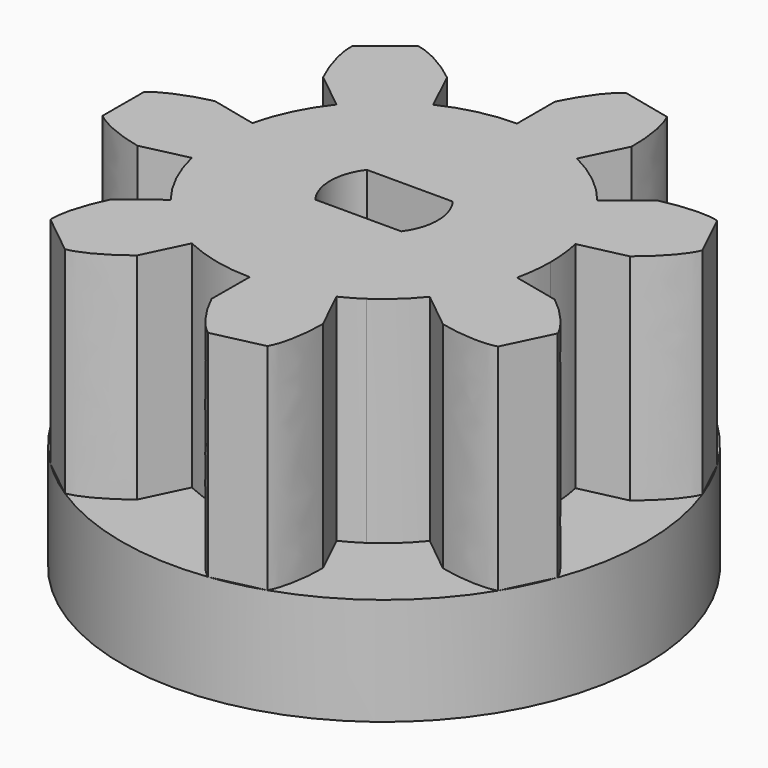
from build123d import *

# Parameters (mm, degrees)
F1_DEPTH        = 10
F2_DEPTH        = 10
F2_COPIES_COUNT = 7
F4_R            = 12.2091154471
F5_DEPTH        = 5


# Not quite as in the source:
# - a pattern or mirror of a feature is missing from the dataset's text; its kind, count and spacing are read off the source's solid


with BuildPart() as f1:
    # F0 (on Top) → F1 (new body)
    with BuildSketch(Plane.XY):
        with BuildLine():
            ThreePointArc((4.3237516011, -6.4317705254), (6.8400137028, -3.6437223475), (7.75, 0))
            ThreePointArc((7.75, 0), (6.5755629687, 4.1017644551), (3.4082008658, 6.9603639889))
            ThreePointArc((3.4082008658, 6.9603639889), (1.7433706712, 7.5513680021), (-0.0120479028, 7.7499906354))
            ThreePointArc((-0.0120479028, 7.7499906354), (-5.6679911875, 5.2854872905), (-7.7319524669, -0.5285934635))
            ThreePointArc((-7.7319524669, -0.5285934635), (-3.4082008658, -6.9603639889), (4.3237516011, -6.4317705254))
        make_face()
        with BuildLine():
            ThreePointArc((-2, -1.5), (-2.5, 0), (-2, 1.5))
            Line((-2, 1.5), (2, 1.5))
            ThreePointArc((2, 1.5), (2.5, 0), (2, -1.5))
            Line((2, -1.5), (-2, -1.5))
        make_face(mode=Mode.SUBTRACT)
    extrude(amount=F1_DEPTH)

    # F0 (on Top) → F2 (join)
    with BuildSketch(Plane.XY):
        with BuildLine():
            ThreePointArc((-0.0120479028, 7.7499906354), (1.7433706712, 7.5513680021), (3.4082008658, 6.9603639889))
            Line((3.4082008658, 6.9603639889), (4.3726173887, 8.9377108908))
            add(Edge.make_bspline(
                [(4.3726173887, 8.9377108908), (4.3837213667, 9.6011226956), (4.2995730436, 10.8287649694), (3.902399388, 11.5686550219)],
                knots=[0, 0, 0, 0, 2.6726339048, 2.6726339048, 2.6726339048, 2.6726339048], degree=3))
            Line((3.902399388, 11.5686550219), (1.5639112325, 12.1085375524))
            add(Edge.make_bspline(
                [(-0.0120479028, 9.9499906354), (0.2687925016, 10.5511288793), (0.8825874647, 11.6176382491), (1.5639112325, 12.1085375524)],
                knots=[0, 0, 0, 0, 2.6726339048, 2.6726339048, 2.6726339048, 2.6726339048], degree=3))
            Line((-0.0120479028, 9.9499906354), (-0.0120479028, 7.7499906354))
        make_face()
    f2 = extrude(amount=F2_DEPTH)

    # F2_copies: F2 ×7 about axis
    f2_copies_axis = Axis((0, 0, 0), (0, 0, 1))
    for i in range(1, F2_COPIES_COUNT):
        add(f2.rotate(f2_copies_axis, i * 360 / F2_COPIES_COUNT))

    # F4 (on face) + F0 (on Top) → F5 (join)
    with BuildSketch(Plane.XY):
        Circle(F4_R)
        with BuildLine():
            ThreePointArc((7.75, 0), (6.8400137028, -3.6437223475), (4.3237516011, -6.4317705254))
            ThreePointArc((4.3237516011, -6.4317705254), (-3.4082008658, -6.9603639889), (-7.7319524669, -0.5285934635))
            ThreePointArc((-7.7319524669, -0.5285934635), (-5.6679911875, 5.2854872905), (-0.0120479028, 7.7499906354))
            ThreePointArc((-0.0120479028, 7.7499906354), (1.7433706712, 7.5513680021), (3.4082008658, 6.9603639889))
            ThreePointArc((3.4082008658, 6.9603639889), (6.5755629687, 4.1017644551), (7.75, 0))
        make_face(mode=Mode.SUBTRACT)
    with BuildSketch(Plane.XY):
        with BuildLine():
            ThreePointArc((4.3237516011, -6.4317705254), (6.8400137028, -3.6437223475), (7.75, 0))
            ThreePointArc((7.75, 0), (6.5755629687, 4.1017644551), (3.4082008658, 6.9603639889))
            ThreePointArc((3.4082008658, 6.9603639889), (1.7433706712, 7.5513680021), (-0.0120479028, 7.7499906354))
            ThreePointArc((-0.0120479028, 7.7499906354), (-5.6679911875, 5.2854872905), (-7.7319524669, -0.5285934635))
            ThreePointArc((-7.7319524669, -0.5285934635), (-3.4082008658, -6.9603639889), (4.3237516011, -6.4317705254))
        make_face()
        with BuildLine():
            ThreePointArc((-2, -1.5), (-2.5, 0), (-2, 1.5))
            Line((-2, 1.5), (2, 1.5))
            ThreePointArc((2, 1.5), (2.5, 0), (2, -1.5))
            Line((2, -1.5), (-2, -1.5))
        make_face(mode=Mode.SUBTRACT)
    extrude(amount=-F5_DEPTH)


solid = f1.part
